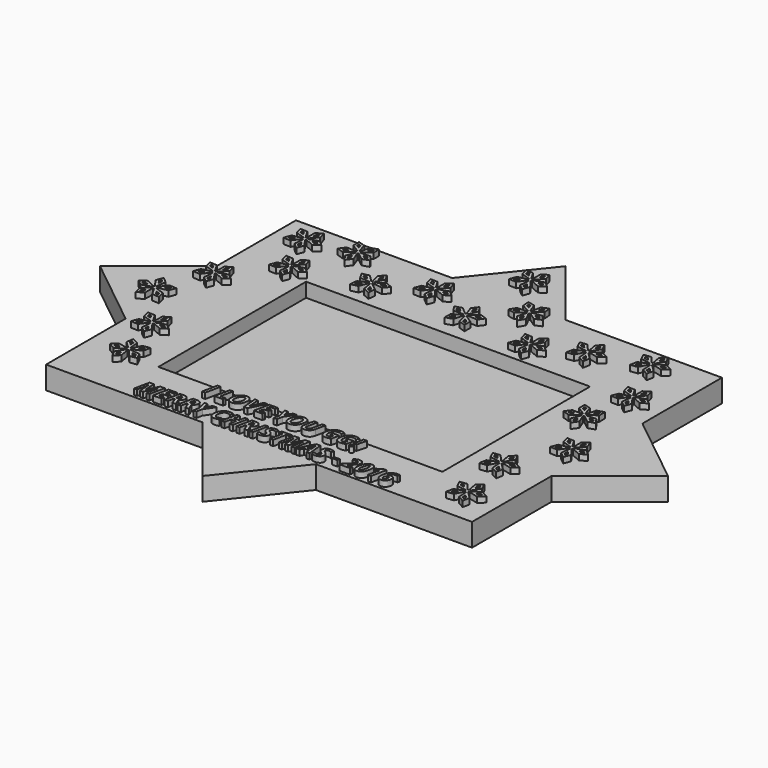
from build123d import *

# Parameters (mm, degrees)
F1_DEPTH     = 4
F4_W         = 100
F4_H         = 65
F5_DEPTH     = 5
F6_DEPTH     = 2
F7_TEXT_SIZE = 7.546576527
F8_DEPTH     = 2


# Not quite as in the source:
# - Text() gives the source's letters only with a copy of the font that has no kerning and outlines rounded to 1/6400 em; it was checked with that copy


with BuildPart() as f1:
    # F0 (on Top) → F1 (new body, symmetric)
    with BuildSketch(Plane.XY):
        Polygon((75, 20), (75, 55), (20, 55), (0, 80), (-20, 55), (-75, 55), (-75, 20), (-100, 0), (-75, -20), (-75, -55), (-20, -55), (0, -80), (20, -55), (75, -55), (75, -20), (100, 0), align=None)
    extrude(amount=F1_DEPTH, both=True)

    # F4 (on face) → F5 (cut)
    with BuildSketch(Plane.XY.offset(4)):
        with Locations((0, -4.2958769202)):
            Rectangle(F4_W, F4_H)
    extrude(amount=-F5_DEPTH, mode=Mode.SUBTRACT)

    # F2 (on face) → F6 (join)
    with BuildSketch(Plane.XY.offset(4)):
        with BuildLine():
            Line((63.1994701679, 31.4178951368), (60.6442793174, 31.5524958216))
            Line((60.6442793174, 31.5524958216), (61.3153708432, 29.0833352779))
            Line((61.3153708432, 29.0833352779), (64.6001066479, 28.016059918))
            ThreePointArc((64.6001066479, 28.016059918), (64.5643629359, 27.8223093015), (64.5803085929, 27.6259355498))
            Line((64.5803085929, 27.6259355498), (61.2044020685, 26.8966748697))
            Line((61.2044020685, 26.8966748697), (60.2867918134, 24.5081378601))
            Line((60.2867918134, 24.5081378601), (62.8424817245, 24.3833712589))
            Line((62.8424817245, 24.3833712589), (64.8725600959, 27.1775344264))
            ThreePointArc((64.8725600959, 27.1775344264), (65.0457824678, 27.083667903), (65.237472483, 27.0381502975))
            Line((65.237472483, 27.0381502975), (64.8878281174, 23.6021184556))
            Line((64.8878281174, 23.6021184556), (66.8759046418, 21.9913207154))
            Line((66.8759046418, 21.9913207154), (67.7843163458, 24.3833712589))
            Line((67.7843163458, 24.3833712589), (65.7542379744, 27.1775344264))
            ThreePointArc((65.7542379744, 27.1775344264), (65.8970389999, 27.313272341), (65.9995642876, 27.4815146655))
            Line((65.9995642876, 27.4815146655), (69.15937871, 26.0871908808))
            Line((69.15937871, 26.0871908808), (71.3056878294, 27.480200138))
            Line((71.3056878294, 27.480200138), (69.3114272272, 29.0833352779))
            Line((69.3114272272, 29.0833352779), (66.0266914224, 28.016059918))
            ThreePointArc((66.0266914224, 28.016059918), (65.9417249379, 28.1938170862), (65.8133990352, 28.3433141666))
            Line((65.8133990352, 28.3433141666), (68.115916112, 30.9176065182))
            Line((68.115916112, 30.9176065182), (67.4543315738, 33.389331326))
            Line((67.4543315738, 33.389331326), (65.3133990352, 31.9880727875))
            Line((65.3133990352, 31.9880727875), (65.3133990352, 28.5342971722))
            ThreePointArc((65.3133990352, 28.5342971722), (65.1180858343, 28.5084192293), (64.9362507771, 28.4325711818))
            Line((64.9362507771, 28.4325711818), (63.1994701679, 31.4178951368))
        make_face()
        Polygon((66.8188202697, 24.1229536578), (66.5160163683, 23.3256034766), (65.8533241935, 23.8625360567), (65.9951811661, 25.2565956289), align=None, mode=Mode.SUBTRACT)
        Polygon((62.2964551725, 25.2211391292), (61.4445585355, 25.2627279962), (61.7504286205, 26.0589069994), (63.1200942761, 26.3547811003), align=None, mode=Mode.SUBTRACT)
        Polygon((61.9434039514, 29.8615218975), (61.7197067761, 30.6845754121), (62.5714370596, 30.6397085171), (63.2760800154, 29.4285091956), align=None, mode=Mode.SUBTRACT)
        Polygon((66.2475713941, 31.6312506978), (66.9612155737, 32.0983368772), (67.1817437531, 31.274428608), (66.2475713941, 30.2299921593), align=None, mode=Mode.SUBTRACT)
        Polygon((69.2607769989, 28.0852630793), (69.9263859742, 27.5501970319), (69.2100289384, 27.0852630793), (67.9263859742, 27.6516931529), align=None, mode=Mode.SUBTRACT)
        with BuildLine():
            Line((60.4743340463, 15.1066376163), (58.0410464334, 15.89798395))
            Line((58.0410464334, 15.89798395), (58.0502052958, 13.3392667437))
            Line((58.0502052958, 13.3392667437), (60.9467852527, 11.4582057254))
            ThreePointArc((60.9467852527, 11.4582057254), (60.8621131286, 11.2803081545), (60.8266901836, 11.0864986364))
            Line((60.8266901836, 11.0864986364), (57.3770683317, 11.2558358144))
            Line((57.3770683317, 11.2558358144), (55.8725260198, 9.1861812398))
            Line((55.8725260198, 9.1861812398), (58.3088409363, 8.404204735))
            Line((58.3088409363, 8.404204735), (60.9929287076, 10.5777361558))
            ThreePointArc((60.9929287076, 10.5777361558), (61.1359542263, 10.4422348077), (61.3093317395, 10.3486551503))
            Line((61.3093317395, 10.3486551503), (60.0822907364, 7.1201978751))
            Line((60.0822907364, 7.1201978751), (61.585720063, 5.0497346693))
            Line((61.585720063, 5.0497346693), (63.0822866263, 7.1251638173))
            Line((63.0822866263, 7.1251638173), (61.8445641408, 10.3495411293))
            ThreePointArc((61.8445641408, 10.3495411293), (62.0176308968, 10.4436942615), (62.1602070378, 10.5796683707))
            Line((62.1602070378, 10.5796683707), (64.8514758442, 8.4150348653))
            Line((64.8514758442, 8.4150348653), (67.2851885796, 9.2050728063))
            Line((67.2851885796, 9.2050728063), (65.7738026656, 11.2697350658))
            Line((65.7738026656, 11.2697350658), (62.3247603297, 11.0889784163))
            ThreePointArc((62.3247603297, 11.0889784163), (62.2886959485, 11.2826696003), (62.2034353365, 11.4602858788))
            Line((62.2034353365, 11.4602858788), (65.0937719348, 13.3509260745))
            Line((65.0937719348, 13.3509260745), (65.0944597975, 15.9096595802))
            Line((65.0944597975, 15.9096595802), (62.6638053693, 15.1102618839))
            Line((62.6638053693, 15.1102618839), (61.7699024625, 11.7741708188))
            ThreePointArc((61.7699024625, 11.7741708188), (61.5745466931, 11.7997254216), (61.379276596, 11.7735242095))
            Line((61.379276596, 11.7735242095), (60.4743340463, 15.1066376163))
        make_face()
        Polygon((62.0822879963, 7.1235085032), (61.5834324752, 6.4316987872), (61.0822893664, 7.1218531892), (61.5801218471, 8.4316960472), align=None, mode=Mode.SUBTRACT)
        Polygon((57.9982500681, 9.3547484281), (57.1861450959, 9.6154072631), (57.6876591999, 10.3052921213), (59.0872324822, 10.2365889995), align=None, mode=Mode.SUBTRACT)
        Polygon((65.4665582086, 10.3187805964), (65.9710018247, 9.6296742031), (65.1587203012, 9.3659893347), (64.0654193012, 10.2453500178), align=None, mode=Mode.SUBTRACT)
        Polygon((58.8582482127, 13.9283903679), (58.8551952585, 14.7812961033), (59.6662911295, 14.5175139921), (60.0334425069, 13.1652102697), align=None, mode=Mode.SUBTRACT)
        Polygon((63.4737942244, 14.5238166141), (64.2840123672, 14.7902825129), (64.2837830796, 13.9373713443), (63.1111218276, 13.1703048025), align=None, mode=Mode.SUBTRACT)
        with BuildLine():
            Line((54.531646123, 49.5059511711), (51.9919011994, 49.1948027344))
            Line((51.9919011994, 49.1948027344), (53.0815625657, 46.879688108))
            Line((53.0815625657, 46.879688108), (56.5017262742, 46.3990154456))
            ThreePointArc((56.5017262742, 46.3990154456), (56.5001700309, 46.2020015058), (56.5499733817, 46.0113800469))
            Line((56.5499733817, 46.0113800469), (53.3519892511, 44.7069784593))
            Line((53.3519892511, 44.7069784593), (52.8630846567, 42.1953873453))
            Line((52.8630846567, 42.1953873453), (55.4016133884, 42.5163071248))
            Line((55.4016133884, 42.5163071248), (56.9156489656, 45.6205400851))
            ThreePointArc((56.9156489656, 45.6205400851), (57.1025394512, 45.5581793543), (57.2992213136, 45.5466398853))
            Line((57.2992213136, 45.5466398853), (57.5515494993, 42.1020939809))
            Line((57.5515494993, 42.1020939809), (59.7891347663, 40.8609937433))
            Line((59.7891347663, 40.8609937433), (60.2683704375, 43.3744477011))
            Line((60.2683704375, 43.3744477011), (57.783932176, 45.773641842))
            ThreePointArc((57.783932176, 45.773641842), (57.9009930915, 45.9321147305), (57.9727458167, 46.1156044054))
            Line((57.9727458167, 46.1156044054), (61.3266773423, 45.2911595482))
            Line((61.3266773423, 45.2911595482), (63.1984856844, 47.035708532))
            Line((63.1984856844, 47.035708532), (60.9561408862, 48.2681887276))
            Line((60.9561408862, 48.2681887276), (57.9066380204, 46.6467392919))
            ThreePointArc((57.9066380204, 46.6467392919), (57.7920951594, 46.8070416542), (57.6397589199, 46.9319839788))
            Line((57.6397589199, 46.9319839788), (59.460274413, 49.8669949397))
            Line((59.460274413, 49.8669949397), (58.3795303219, 52.1862857442))
            Line((58.3795303219, 52.1862857442), (56.5144493508, 50.4345464378))
            Line((56.5144493508, 50.4345464378), (57.1141911925, 47.0332414346))
            ThreePointArc((57.1141911925, 47.0332414346), (56.9263388957, 46.9738408544), (56.7604371968, 46.8675697828))
            Line((56.7604371968, 46.8675697828), (54.531646123, 49.5059511711))
        make_face()
        Polygon((54.7184053426, 43.246530903), (53.8722290987, 43.1395576431), (54.0351972969, 43.9767546812), (55.3326766551, 44.5059737347), align=None, mode=Mode.SUBTRACT)
        Polygon((53.5649237515, 47.755109129), (53.201703296, 48.5268140045), (54.0482849372, 48.6305301501), (54.9525453381, 47.560091633), align=None, mode=Mode.SUBTRACT)
        Polygon((59.3627634581, 42.9503297944), (59.2030182344, 42.1125118084), (58.4571564787, 42.5262118876), (58.3547824209, 43.9237257673), align=None, mode=Mode.SUBTRACT)
        Polygon((61.0795735671, 47.2764841685), (61.8279836906, 46.8651287623), (61.2032446614, 46.2828641073), (59.8407435681, 46.6177865738), align=None, mode=Mode.SUBTRACT)
        Polygon((57.4963910382, 50.2453626051), (58.1180846952, 50.8292757072), (58.4783327256, 50.0561787724), (57.7397170299, 48.8653923324), align=None, mode=Mode.SUBTRACT)
        with BuildLine():
            Line((69.176194365, -2.7749478988), (66.6210035146, -2.640347214))
            Line((66.6210035146, -2.640347214), (67.2920950403, -5.1095077577))
            Line((67.2920950403, -5.1095077577), (70.5768308451, -6.1767831176))
            ThreePointArc((70.5768308451, -6.1767831176), (70.5410871331, -6.3705337341), (70.5570327901, -6.5669074858))
            Line((70.5570327901, -6.5669074858), (67.1811262657, -7.2961681658))
            Line((67.1811262657, -7.2961681658), (66.2635160106, -9.6847051755))
            Line((66.2635160106, -9.6847051755), (68.8192059217, -9.8094717767))
            Line((68.8192059217, -9.8094717767), (70.8492842931, -7.0153086091))
            ThreePointArc((70.8492842931, -7.0153086091), (71.022506665, -7.1091751326), (71.2141966802, -7.1546927381))
            Line((71.2141966802, -7.1546927381), (70.8645523146, -10.59072458))
            Line((70.8645523146, -10.59072458), (72.852628839, -12.2015223202))
            Line((72.852628839, -12.2015223202), (73.761040543, -9.8094717767))
            Line((73.761040543, -9.8094717767), (71.7309621716, -7.0153086091))
            ThreePointArc((71.7309621716, -7.0153086091), (71.8737631971, -6.8795706945), (71.9762884848, -6.7113283701))
            Line((71.9762884848, -6.7113283701), (75.1361029072, -8.1056521548))
            Line((75.1361029072, -8.1056521548), (77.2824120266, -6.7126428976))
            Line((77.2824120266, -6.7126428976), (75.2881514244, -5.1095077577))
            Line((75.2881514244, -5.1095077577), (72.0034156196, -6.1767831176))
            ThreePointArc((72.0034156196, -6.1767831176), (71.9184491351, -5.9990259494), (71.7901232323, -5.849528869))
            Line((71.7901232323, -5.849528869), (74.0926403092, -3.2752365174))
            Line((74.0926403092, -3.2752365174), (73.431055771, -0.8035117096))
            Line((73.431055771, -0.8035117096), (71.2901232323, -2.204770248))
            Line((71.2901232323, -2.204770248), (71.2901232323, -5.6585458634))
            ThreePointArc((71.2901232323, -5.6585458634), (71.0948100315, -5.6844238063), (70.9129749743, -5.7602718538))
            Line((70.9129749743, -5.7602718538), (69.176194365, -2.7749478988))
        make_face()
        Polygon((72.7955444668, -10.0698893778), (72.4927405655, -10.867239559), (71.8300483907, -10.3303069789), (71.9719053633, -8.9362474067), align=None, mode=Mode.SUBTRACT)
        Polygon((68.2731793697, -8.9717039064), (67.4212827327, -8.9301150393), (67.7271528177, -8.1339360361), (69.0968184732, -7.8380619353), align=None, mode=Mode.SUBTRACT)
        Polygon((75.237501196, -6.1075799563), (75.9031101714, -6.6426460036), (75.1867531355, -7.1075799563), (73.9031101714, -6.5411498826), align=None, mode=Mode.SUBTRACT)
        Polygon((67.9201281486, -4.3313211381), (67.6964309733, -3.5082676235), (68.5481612568, -3.5531345184), (69.2528042126, -4.76433384), align=None, mode=Mode.SUBTRACT)
        Polygon((72.2242955913, -2.5615923378), (72.9379397709, -2.0945061583), (73.1584679503, -2.9184144276), (72.2242955913, -3.9628508763), align=None, mode=Mode.SUBTRACT)
        with BuildLine():
            Line((58.7020704823, -22.0312884666), (56.1623255587, -22.3424369034))
            Line((56.1623255587, -22.3424369034), (57.2519869251, -24.6575515297))
            Line((57.2519869251, -24.6575515297), (60.6721506335, -25.1382241921))
            ThreePointArc((60.6721506335, -25.1382241921), (60.6705943902, -25.3352381319), (60.720397741, -25.5258595908))
            Line((60.720397741, -25.5258595908), (57.5224136105, -26.8302611784))
            Line((57.5224136105, -26.8302611784), (57.033509016, -29.3418522924))
            Line((57.033509016, -29.3418522924), (59.5720377477, -29.0209325129))
            Line((59.5720377477, -29.0209325129), (61.086073325, -25.9166995526))
            ThreePointArc((61.086073325, -25.9166995526), (61.2729638106, -25.9790602834), (61.469645673, -25.9905997524))
            Line((61.469645673, -25.9905997524), (61.7219738586, -29.4351456568))
            Line((61.7219738586, -29.4351456568), (63.9595591256, -30.6762458944))
            Line((63.9595591256, -30.6762458944), (64.4387947969, -28.1627919366))
            Line((64.4387947969, -28.1627919366), (61.9543565353, -25.7635977957))
            ThreePointArc((61.9543565353, -25.7635977957), (62.0714174509, -25.6051249072), (62.143170176, -25.4216352323))
            Line((62.143170176, -25.4216352323), (65.4971017016, -26.2460800895))
            Line((65.4971017016, -26.2460800895), (67.3689100438, -24.5015311057))
            Line((67.3689100438, -24.5015311057), (65.1265652456, -23.2690509101))
            Line((65.1265652456, -23.2690509101), (62.0770623797, -24.8905003458))
            ThreePointArc((62.0770623797, -24.8905003458), (61.9625195187, -24.7301979835), (61.8101832792, -24.6052556589))
            Line((61.8101832792, -24.6052556589), (63.6306987723, -21.670244698))
            Line((63.6306987723, -21.670244698), (62.5499546812, -19.3509538935))
            Line((62.5499546812, -19.3509538935), (60.6848737102, -21.1026932))
            Line((60.6848737102, -21.1026932), (61.2846155518, -24.5039982031))
            ThreePointArc((61.2846155518, -24.5039982031), (61.096763255, -24.5633987833), (60.9308615561, -24.6696698549))
            Line((60.9308615561, -24.6696698549), (58.7020704823, -22.0312884666))
        make_face()
        Polygon((58.888829702, -28.2907087347), (58.0426534581, -28.3976819946), (58.2056216562, -27.5604849566), (59.5031010144, -27.031265903), align=None, mode=Mode.SUBTRACT)
        Polygon((63.5331878175, -28.5869098433), (63.3734425937, -29.4247278293), (62.627580838, -29.0110277501), (62.5252067802, -27.6135138704), align=None, mode=Mode.SUBTRACT)
        Polygon((65.2499979265, -24.2607554692), (65.99840805, -24.6721108754), (65.3736690207, -25.2543755304), (64.0111679275, -24.9194530639), align=None, mode=Mode.SUBTRACT)
        Polygon((57.7353481108, -23.7821305087), (57.3721276554, -23.0104256332), (58.2187092966, -22.9067094876), (59.1229696975, -23.9771480047), align=None, mode=Mode.SUBTRACT)
        Polygon((61.6668153975, -21.2918770327), (62.2885090546, -20.7079639305), (62.6487570849, -21.4810608653), (61.9101413892, -22.6718473053), align=None, mode=Mode.SUBTRACT)
        with BuildLine():
            Line((62.2558930258, -41.1344152125), (59.7161481023, -41.4455636493))
            Line((59.7161481023, -41.4455636493), (60.8058094686, -43.7606782757))
            Line((60.8058094686, -43.7606782757), (64.225973177, -44.2413509381))
            ThreePointArc((64.225973177, -44.2413509381), (64.2244169338, -44.4383648779), (64.2742202845, -44.6289863368))
            Line((64.2742202845, -44.6289863368), (61.076236154, -45.9333879244))
            Line((61.076236154, -45.9333879244), (60.5873315596, -48.4449790384))
            Line((60.5873315596, -48.4449790384), (63.1258602913, -48.1240592589))
            Line((63.1258602913, -48.1240592589), (64.6398958685, -45.0198262986))
            ThreePointArc((64.6398958685, -45.0198262986), (64.8267863541, -45.0821870294), (65.0234682165, -45.0937264984))
            Line((65.0234682165, -45.0937264984), (65.2757964021, -48.5382724028))
            Line((65.2757964021, -48.5382724028), (67.5133816691, -49.7793726404))
            Line((67.5133816691, -49.7793726404), (67.9926173404, -47.2659186826))
            Line((67.9926173404, -47.2659186826), (65.5081790789, -44.8667245417))
            ThreePointArc((65.5081790789, -44.8667245417), (65.6252399944, -44.7082516532), (65.6969927195, -44.5247619783))
            Line((65.6969927195, -44.5247619783), (69.0509242452, -45.3492068355))
            Line((69.0509242452, -45.3492068355), (70.9227325873, -43.6046578517))
            Line((70.9227325873, -43.6046578517), (68.6803877891, -42.3721776561))
            Line((68.6803877891, -42.3721776561), (65.6308849232, -43.9936270918))
            ThreePointArc((65.6308849232, -43.9936270918), (65.5163420622, -43.8333247295), (65.3640058227, -43.7083824049))
            Line((65.3640058227, -43.7083824049), (67.1845213159, -40.773371444))
            Line((67.1845213159, -40.773371444), (66.1037772248, -38.4540806395))
            Line((66.1037772248, -38.4540806395), (64.2386962537, -40.2058199459))
            Line((64.2386962537, -40.2058199459), (64.8384380953, -43.6071249491))
            ThreePointArc((64.8384380953, -43.6071249491), (64.6505857985, -43.6665255293), (64.4846840997, -43.7727966009))
            Line((64.4846840997, -43.7727966009), (62.2558930258, -41.1344152125))
        make_face()
        Polygon((62.4426522455, -47.3938354807), (61.5964760016, -47.5008087405), (61.7594441997, -46.6636117025), (63.0569235579, -46.134392649), align=None, mode=Mode.SUBTRACT)
        Polygon((67.087010361, -47.6900365893), (66.9272651372, -48.5278545752), (66.1814033816, -48.1141544961), (66.0790293237, -46.7166406164), align=None, mode=Mode.SUBTRACT)
        Polygon((61.2891706543, -42.8852572547), (60.9259501989, -42.1135523792), (61.7725318401, -42.0098362336), (62.676792241, -43.0802747507), align=None, mode=Mode.SUBTRACT)
        Polygon((68.80382047, -43.3638822152), (69.5522305935, -43.7752376214), (68.9274915642, -44.3575022764), (67.564990471, -44.0225798099), align=None, mode=Mode.SUBTRACT)
        Polygon((65.2206379411, -40.3950037786), (65.8423315981, -39.8110906765), (66.2025796285, -40.5841876113), (65.4639639327, -41.7749740513), align=None, mode=Mode.SUBTRACT)
        with BuildLine():
            Line((36.2130666452, 44.3193224602), (33.6733217216, 44.0081740234))
            Line((33.6733217216, 44.0081740234), (34.7629830879, 41.693059397))
            Line((34.7629830879, 41.693059397), (38.1831467964, 41.2123867346))
            ThreePointArc((38.1831467964, 41.2123867346), (38.1815905531, 41.0153727949), (38.2313939039, 40.824751336))
            Line((38.2313939039, 40.824751336), (35.0334097734, 39.5203497484))
            Line((35.0334097734, 39.5203497484), (34.5445051789, 37.0087586343))
            Line((34.5445051789, 37.0087586343), (37.0830339106, 37.3296784138))
            Line((37.0830339106, 37.3296784138), (38.5970694879, 40.4339113742))
            ThreePointArc((38.5970694879, 40.4339113742), (38.7839599734, 40.3715506433), (38.9806418359, 40.3600111743))
            Line((38.9806418359, 40.3600111743), (39.2329700215, 36.9154652699))
            Line((39.2329700215, 36.9154652699), (41.4705552885, 35.6743650324))
            Line((41.4705552885, 35.6743650324), (41.9497909598, 38.1878189902))
            Line((41.9497909598, 38.1878189902), (39.4653526982, 40.587013131))
            ThreePointArc((39.4653526982, 40.587013131), (39.5824136138, 40.7454860196), (39.6541663389, 40.9289756944))
            Line((39.6541663389, 40.9289756944), (43.0080978645, 40.1045308373))
            Line((43.0080978645, 40.1045308373), (44.8799062067, 41.8490798211))
            Line((44.8799062067, 41.8490798211), (42.6375614084, 43.0815600166))
            Line((42.6375614084, 43.0815600166), (39.5880585426, 41.460110581))
            ThreePointArc((39.5880585426, 41.460110581), (39.4735156816, 41.6204129432), (39.3211794421, 41.7453552678))
            Line((39.3211794421, 41.7453552678), (41.1416949352, 44.6803662287))
            Line((41.1416949352, 44.6803662287), (40.0609508441, 46.9996570333))
            Line((40.0609508441, 46.9996570333), (38.195869873, 45.2479177268))
            Line((38.195869873, 45.2479177268), (38.7956117147, 41.8466127236))
            ThreePointArc((38.7956117147, 41.8466127236), (38.6077594179, 41.7872121434), (38.441857719, 41.6809410719))
            Line((38.441857719, 41.6809410719), (36.2130666452, 44.3193224602))
        make_face()
        Polygon((36.3998258649, 38.059902192), (35.553649621, 37.9529289322), (35.7166178191, 38.7901259702), (37.0140971773, 39.3193450237), align=None, mode=Mode.SUBTRACT)
        Polygon((41.0441839804, 37.7637010834), (40.8844387566, 36.9258830975), (40.1385770009, 37.3395831767), (40.0362029431, 38.7370970563), align=None, mode=Mode.SUBTRACT)
        Polygon((35.2463442737, 42.5684804181), (34.8831238183, 43.3401852935), (35.7297054595, 43.4439014391), (36.6339658604, 42.373462922), align=None, mode=Mode.SUBTRACT)
        Polygon((42.7609940894, 42.0898554576), (43.5094042129, 41.6785000513), (42.8846651836, 41.0962353963), (41.5221640904, 41.4311578629), align=None, mode=Mode.SUBTRACT)
        Polygon((39.1778115604, 45.0587338941), (39.7995052175, 45.6426469963), (40.1597532478, 44.8695500614), (39.4211375521, 43.6787636215), align=None, mode=Mode.SUBTRACT)
        with BuildLine():
            Line((-2.0873219995, 68.2391146027), (-4.6425128499, 68.3737152875))
            Line((-4.6425128499, 68.3737152875), (-3.9714213242, 65.9045547438))
            Line((-3.9714213242, 65.9045547438), (-0.6866855194, 64.8372793839))
            ThreePointArc((-0.6866855194, 64.8372793839), (-0.7224292314, 64.6435287674), (-0.7064835744, 64.4471550157))
            Line((-0.7064835744, 64.4471550157), (-4.0823900988, 63.7178943357))
            Line((-4.0823900988, 63.7178943357), (-5.0000003539, 61.329357326))
            Line((-5.0000003539, 61.329357326), (-2.4443104428, 61.2045907248))
            Line((-2.4443104428, 61.2045907248), (-0.4142320714, 63.9987538923))
            ThreePointArc((-0.4142320714, 63.9987538923), (-0.2410096995, 63.9048873689), (-0.0493196843, 63.8593697634))
            Line((-0.0493196843, 63.8593697634), (-0.3989640499, 60.4233379215))
            Line((-0.3989640499, 60.4233379215), (1.5891124745, 58.8125401813))
            Line((1.5891124745, 58.8125401813), (2.4975241785, 61.2045907248))
            Line((2.4975241785, 61.2045907248), (0.4674458071, 63.9987538923))
            ThreePointArc((0.4674458071, 63.9987538923), (0.6102468326, 64.1344918069), (0.7127721203, 64.3027341314))
            Line((0.7127721203, 64.3027341314), (3.8725865427, 62.9084103467))
            Line((3.8725865427, 62.9084103467), (6.0188956621, 64.3014196039))
            Line((6.0188956621, 64.3014196039), (4.0246350599, 65.9045547438))
            Line((4.0246350599, 65.9045547438), (0.7398992551, 64.8372793839))
            ThreePointArc((0.7398992551, 64.8372793839), (0.6549327706, 65.0150365521), (0.5266068679, 65.1645336325))
            Line((0.5266068679, 65.1645336325), (2.8291239447, 67.7388259841))
            Line((2.8291239447, 67.7388259841), (2.1675394065, 70.2105507919))
            Line((2.1675394065, 70.2105507919), (0.0266068679, 68.8092922535))
            Line((0.0266068679, 68.8092922535), (0.0266068679, 65.3555166381))
            ThreePointArc((0.0266068679, 65.3555166381), (-0.168706333, 65.3296386952), (-0.3505413902, 65.2537906477))
            Line((-0.3505413902, 65.2537906477), (-2.0873219995, 68.2391146027))
        make_face()
        Polygon((-2.9903369948, 62.0423585951), (-3.8422336318, 62.0839474622), (-3.5363635468, 62.8801264654), (-2.1666978913, 63.1760005662), align=None, mode=Mode.SUBTRACT)
        Polygon((1.5320281024, 60.9441731237), (1.229224201, 60.1468229425), (0.5665320262, 60.6837555226), (0.7083889988, 62.0778150948), align=None, mode=Mode.SUBTRACT)
        Polygon((3.9739848315, 64.9064825452), (4.6395938069, 64.3714164979), (3.923236771, 63.9064825452), (2.6395938069, 64.4729126189), align=None, mode=Mode.SUBTRACT)
        Polygon((-3.3433882159, 66.6827413634), (-3.5670853912, 67.505794878), (-2.7153551077, 67.4609279831), (-2.0107121519, 66.2497286615), align=None, mode=Mode.SUBTRACT)
        Polygon((0.9607792268, 68.4524701637), (1.6744234064, 68.9195563432), (1.8949515858, 68.0956480739), (0.9607792268, 67.0512116252), align=None, mode=Mode.SUBTRACT)
        with BuildLine():
            Line((10.203743278, 53.3324640832), (7.7107446817, 53.908724116))
            Line((7.7107446817, 53.908724116), (7.9428755905, 51.3605418486))
            Line((7.9428755905, 51.3605418486), (10.9923784563, 49.7390924129))
            ThreePointArc((10.9923784563, 49.7390924129), (10.9235333301, 49.5544921341), (10.9051367926, 49.3583328066))
            Line((10.9051367926, 49.3583328066), (7.4538830858, 49.2263712509))
            Line((7.4538830858, 49.2263712509), (6.1354482933, 47.0334628341))
            Line((6.1354482933, 47.0334628341), (8.6306460392, 46.4668008221))
            Line((8.6306460392, 46.4668008221), (11.1150843007, 48.865994963))
            ThreePointArc((11.1150843007, 48.865994963), (11.2693752848, 48.7434747338), (11.4502490487, 48.6653620211))
            Line((11.4502490487, 48.6653620211), (10.5092558989, 45.3422463305))
            Line((10.5092558989, 45.3422463305), (12.1874169815, 43.410694362))
            Line((12.1874169815, 43.410694362), (13.4974030883, 45.6086602458))
            Line((13.4974030883, 45.6086602458), (11.9833675111, 48.7128932061))
            ThreePointArc((11.9833675111, 48.7128932061), (12.1475697096, 48.821771819), (12.2777523809, 48.9696548351))
            Line((12.2777523809, 48.9696548351), (15.1474403379, 47.0478179455))
            Line((15.1474403379, 47.0478179455), (17.503035718, 48.0469615947))
            Line((17.503035718, 48.0469615947), (15.817453911, 49.972041229))
            Line((15.817453911, 49.972041229), (12.3972902025, 49.4913685666))
            ThreePointArc((12.3972902025, 49.4913685666), (12.3444817582, 49.6811794792), (12.2440653098, 49.8506889221))
            Line((12.2440653098, 49.8506889221), (14.9586231542, 51.9860440941))
            Line((14.9586231542, 51.9860440941), (14.7363000803, 54.5351007975))
            Line((14.7363000803, 54.5351007975), (12.3845671259, 53.5268995588))
            Line((12.3845671259, 53.5268995588), (11.7848252842, 50.1255945556))
            ThreePointArc((11.7848252842, 50.1255945556), (11.5879856721, 50.1340255382), (11.3957422228, 50.0909051192))
            Line((11.3957422228, 50.0909051192), (10.203743278, 53.3324640832))
        make_face()
        Polygon((12.5013540252, 45.5198556074), (12.0646919895, 44.7872003128), (11.505304962, 45.431050969), (11.8870827127, 46.7792984391), align=None, mode=Mode.SUBTRACT)
        Polygon((8.2383917214, 47.3866576317), (7.4066591394, 47.5755449691), (7.8461374036, 48.3065144413), (9.2463727586, 48.3600536046), align=None, mode=Mode.SUBTRACT)
        Polygon((15.594259755, 48.9979273096), (16.1568433904, 48.3554083322), (15.3706344939, 48.0219318648), (14.2048525008, 48.8026588544), align=None, mode=Mode.SUBTRACT)
        Polygon((8.696498153, 52.0178492601), (8.6191211834, 52.8672433492), (9.4501207155, 52.6751566717), (9.9337360065, 51.3599982242), align=None, mode=Mode.SUBTRACT)
        Polygon((13.242585802, 53.0132810705), (14.0264967868, 53.3493481501), (14.1006044781, 52.4996625823), (12.9992598104, 51.6333107979), align=None, mode=Mode.SUBTRACT)
        with BuildLine():
            Line((-4.2115295507, 39.8939389404), (-6.6586596831, 39.1464954698))
            Line((-6.6586596831, 39.1464954698), (-5.1835372855, 37.0557703471))
            Line((-5.1835372855, 37.0557703471), (-1.7318656169, 37.1763053778))
            ThreePointArc((-1.7318656169, 37.1763053778), (-1.6991871057, 36.9820142837), (-1.6170393108, 36.8029370542))
            Line((-1.6170393108, 36.8029370542), (-4.539931918, 34.9630281412))
            Line((-4.539931918, 34.9630281412), (-4.585275733, 32.4046963479))
            Line((-4.585275733, 32.4046963479), (-2.1410400917, 33.161551523))
            Line((-2.1410400917, 33.161551523), (-1.1890505135, 36.4815337284))
            ThreePointArc((-1.1890505135, 36.4815337284), (-0.9941704871, 36.4525735895), (-0.7984728563, 36.4753628779))
            Line((-0.7984728563, 36.4753628779), (0.0481610164, 33.1269636952))
            Line((0.0481610164, 33.1269636952), (2.4672671299, 32.293271163))
            Line((2.4672671299, 32.293271163), (2.5027654351, 34.8517585085))
            Line((2.5027654351, 34.8517585085), (-0.3605443172, 36.7830853228))
            ThreePointArc((-0.3605443172, 36.7830853228), (-0.2727803483, 36.9594780667), (-0.233980356, 37.1526398511))
            Line((-0.233980356, 37.1526398511), (3.2121607606, 36.9231242612))
            Line((3.2121607606, 36.9231242612), (4.7525943762, 38.9662057335))
            Line((4.7525943762, 38.9662057335), (2.330297894, 39.7905826976))
            Line((2.330297894, 39.7905826976), (-0.3913144314, 37.6642261069))
            ThreePointArc((-0.3913144314, 37.6642261069), (-0.5319533421, 37.8022029569), (-0.7036712588, 37.8987942165))
            Line((-0.7036712588, 37.8987942165), (0.5795272085, 41.1053449638))
            Line((0.5795272085, 41.1053449638), (-0.8875385731, 43.2017312876))
            Line((-0.8875385731, 43.2017312876), (-2.4200984351, 41.1527369255))
            Line((-2.4200984351, 41.1527369255), (-1.2388376041, 37.907249466))
            ThreePointArc((-1.2388376041, 37.907249466), (-1.4135212, 37.816131105), (-1.5584487013, 37.6826660021))
            Line((-1.5584487013, 37.6826660021), (-4.2115295507, 39.8939389404))
        make_face()
        Polygon((-4.8595347072, 38.0018265449), (-5.3512421731, 38.6987349191), (-4.535532129, 38.9478827426), (-3.4591297776, 38.0507297626), align=None, mode=Mode.SUBTRACT)
        Polygon((-2.9406707005, 33.7620437291), (-3.7554159142, 33.5097586707), (-3.7403013092, 34.3625359352), (-2.5544315021, 35.1090198882), align=None, mode=Mode.SUBTRACT)
        Polygon((1.6845639622, 34.2768269041), (1.6727311938, 33.4239977889), (0.8663624893, 33.7018952997), (0.5228679849, 35.0604007347), align=None, mode=Mode.SUBTRACT)
        Polygon((2.6240630446, 38.8353782193), (3.4325342533, 38.5602322801), (2.91839561, 37.8783287396), (1.5184352939, 37.9715671494), align=None, mode=Mode.SUBTRACT)
        Polygon((-1.4202232206, 41.1369396049), (-0.9093699332, 41.8199377256), (-0.420348006, 41.1211422844), (-0.9409645744, 39.8201872966), align=None, mode=Mode.SUBTRACT)
        with BuildLine():
            Line((-19.2796059392, 47.6930219819), (-21.8347967896, 47.8276226667))
            Line((-21.8347967896, 47.8276226667), (-21.1637052639, 45.358462123))
            Line((-21.1637052639, 45.358462123), (-17.8789694591, 44.2911867631))
            ThreePointArc((-17.8789694591, 44.2911867631), (-17.9147131711, 44.0974361466), (-17.8987675141, 43.9010623949))
            Line((-17.8987675141, 43.9010623949), (-21.2746740385, 43.1718017149))
            Line((-21.2746740385, 43.1718017149), (-22.1922842936, 40.7832647052))
            Line((-22.1922842936, 40.7832647052), (-19.6365943825, 40.658498104))
            Line((-19.6365943825, 40.658498104), (-17.6065160111, 43.4526612716))
            ThreePointArc((-17.6065160111, 43.4526612716), (-17.4332936392, 43.3587947481), (-17.241603624, 43.3132771426))
            Line((-17.241603624, 43.3132771426), (-17.5912479896, 39.8772453007))
            Line((-17.5912479896, 39.8772453007), (-15.6031714652, 38.2664475605))
            Line((-15.6031714652, 38.2664475605), (-14.6947597612, 40.658498104))
            Line((-14.6947597612, 40.658498104), (-16.7248381326, 43.4526612716))
            ThreePointArc((-16.7248381326, 43.4526612716), (-16.5820371071, 43.5883991862), (-16.4795118194, 43.7566415106))
            Line((-16.4795118194, 43.7566415106), (-13.319697397, 42.3623177259))
            Line((-13.319697397, 42.3623177259), (-11.1733882776, 43.7553269831))
            Line((-11.1733882776, 43.7553269831), (-13.1676488798, 45.358462123))
            Line((-13.1676488798, 45.358462123), (-16.4523846846, 44.2911867631))
            ThreePointArc((-16.4523846846, 44.2911867631), (-16.5373511691, 44.4689439313), (-16.6656770719, 44.6184410117))
            Line((-16.6656770719, 44.6184410117), (-14.363159995, 47.1927333633))
            Line((-14.363159995, 47.1927333633), (-15.0247445332, 49.6644581711))
            Line((-15.0247445332, 49.6644581711), (-17.1656770719, 48.2631996327))
            Line((-17.1656770719, 48.2631996327), (-17.1656770719, 44.8094240173))
            ThreePointArc((-17.1656770719, 44.8094240173), (-17.3609902727, 44.7835460744), (-17.5428253299, 44.7076980269))
            Line((-17.5428253299, 44.7076980269), (-19.2796059392, 47.6930219819))
        make_face()
        Polygon((-20.1826209345, 41.4962659743), (-21.0345175715, 41.5378548414), (-20.7286474865, 42.3340338446), (-19.358981831, 42.6299079454), align=None, mode=Mode.SUBTRACT)
        Polygon((-15.6602558374, 40.3980805029), (-15.9630597387, 39.6007303217), (-16.6257519135, 40.1376629018), (-16.4838949409, 41.531722474), align=None, mode=Mode.SUBTRACT)
        Polygon((-13.2182991082, 44.3603899244), (-12.5526901328, 43.8253238771), (-13.2690471687, 43.3603899244), (-14.5526901328, 43.9268199981), align=None, mode=Mode.SUBTRACT)
        Polygon((-20.5356721556, 46.1366487426), (-20.7593693309, 46.9597022572), (-19.9076390474, 46.9148353623), (-19.2029960916, 45.7036360407), align=None, mode=Mode.SUBTRACT)
        Polygon((-16.2315047129, 47.9063775429), (-15.5178605333, 48.3734637224), (-15.2973323539, 47.5495554531), (-16.2315047129, 46.5051190045), align=None, mode=Mode.SUBTRACT)
        with BuildLine():
            Line((-36.2098404653, 39.0344415003), (-38.7128025196, 38.503123722))
            Line((-38.7128025196, 38.503123722), (-37.4255121089, 36.2917890515))
            Line((-37.4255121089, 36.2917890515), (-33.976469773, 36.111032402))
            ThreePointArc((-33.976469773, 36.111032402), (-33.9608491981, 35.9146325242), (-33.8946216093, 35.7290770856))
            Line((-33.8946216093, 35.7290770856), (-36.9667503555, 34.1509164576))
            Line((-36.9667503555, 34.1509164576), (-37.2348949313, 31.606271863))
            Line((-37.2348949313, 31.606271863), (-34.7339960696, 32.147217803))
            Line((-34.7339960696, 32.147217803), (-33.4962735841, 35.3715951149))
            ThreePointArc((-33.4962735841, 35.3715951149), (-33.3046591775, 35.3257602646), (-33.1077200179, 35.3314066606))
            Line((-33.1077200179, 35.3314066606), (-32.5561400605, 31.9219601437))
            Line((-32.5561400605, 31.9219601437), (-30.218900468, 30.8806010732))
            Line((-30.218900468, 30.8806010732), (-29.9605503796, 33.4262587207))
            Line((-29.9605503796, 33.4262587207), (-32.6446381509, 35.5997901415))
            ThreePointArc((-32.6446381509, 35.5997901415), (-32.5418345098, 35.7678625239), (-32.4863470043, 35.9569076272))
            Line((-32.4863470043, 35.9569076272), (-29.0733230968, 35.4279144249))
            Line((-29.0733230968, 35.4279144249), (-27.360685013, 37.3289637194))
            Line((-27.360685013, 37.3289637194), (-29.7019147391, 38.3613207294))
            Line((-29.7019147391, 38.3613207294), (-32.598494696, 36.4802597111))
            ThreePointArc((-32.598494696, 36.4802597111), (-32.7265729583, 36.6299690063), (-32.8892189535, 36.7411589096))
            Line((-32.8892189535, 36.7411589096), (-31.3314341317, 39.8236696476))
            Line((-31.3314341317, 39.8236696476), (-32.610205178, 42.0399417965))
            Line((-32.610205178, 42.0399417965), (-34.3155148126, 40.1323158696))
            Line((-34.3155148126, 40.1323158696), (-33.4216119058, 36.7962248045))
            ThreePointArc((-33.4216119058, 36.7962248045), (-33.6035722662, 36.720677855), (-33.7595805249, 36.6003518911))
            Line((-33.7595805249, 36.6003518911), (-36.2098404653, 39.0344415003))
        make_face()
        Polygon((-35.4782474982, 32.8151173545), (-36.3118804521, 32.6348020412), (-36.2224989269, 33.4830169061), (-34.976081349, 34.1233048985), align=None, mode=Mode.SUBTRACT)
        Polygon((-37.0202882277, 37.2060065344), (-37.4493850313, 37.9431180913), (-36.6150643465, 38.1202240173), (-35.6209500654, 37.1326703289), align=None, mode=Mode.SUBTRACT)
        Polygon((-30.8257469399, 32.9248258617), (-30.911863636, 32.0762733125), (-31.6909435002, 32.4233930027), (-31.914729354, 33.8066664331), align=None, mode=Mode.SUBTRACT)
        Polygon((-29.4925190094, 37.3841477725), (-28.7111048264, 37.039585938), (-29.2827188266, 36.4050873817), (-30.6692256081, 36.6199855724), align=None, mode=Mode.SUBTRACT)
        Polygon((-33.3208212523, 40.0294337956), (-32.7523847074, 40.6653091045), (-32.326127692, 39.9265517216), (-32.9581488554, 38.675921984), align=None, mode=Mode.SUBTRACT)
        with BuildLine():
            Line((-48.5238044113, 51.9647017388), (-50.9570920241, 52.7560480725))
            Line((-50.9570920241, 52.7560480725), (-50.9479331617, 50.1973308662))
            Line((-50.9479331617, 50.1973308662), (-48.0513532048, 48.3162698479))
            ThreePointArc((-48.0513532048, 48.3162698479), (-48.136025329, 48.138372277), (-48.171448274, 47.9445627589))
            Line((-48.171448274, 47.9445627589), (-51.6210701259, 48.1138999369))
            Line((-51.6210701259, 48.1138999369), (-53.1256124377, 46.0442453623))
            Line((-53.1256124377, 46.0442453623), (-50.6892975212, 45.2622688575))
            Line((-50.6892975212, 45.2622688575), (-48.00520975, 47.4358002783))
            ThreePointArc((-48.00520975, 47.4358002783), (-47.8621842312, 47.3002989302), (-47.6888067181, 47.2067192728))
            Line((-47.6888067181, 47.2067192728), (-48.9158477211, 43.9782619976))
            Line((-48.9158477211, 43.9782619976), (-47.4124183946, 41.9077987918))
            Line((-47.4124183946, 41.9077987918), (-45.9158518312, 43.9832279398))
            Line((-45.9158518312, 43.9832279398), (-47.1535743167, 47.2076052518))
            ThreePointArc((-47.1535743167, 47.2076052518), (-46.9805075607, 47.301758384), (-46.8379314197, 47.4377324932))
            Line((-46.8379314197, 47.4377324932), (-44.1466626133, 45.2730989878))
            Line((-44.1466626133, 45.2730989878), (-41.7129498779, 46.0631369288))
            Line((-41.7129498779, 46.0631369288), (-43.2243357919, 48.1277991883))
            Line((-43.2243357919, 48.1277991883), (-46.6733781278, 47.9470425388))
            ThreePointArc((-46.6733781278, 47.9470425388), (-46.709442509, 48.1407337228), (-46.794703121, 48.3183500013))
            Line((-46.794703121, 48.3183500013), (-43.9043665227, 50.208990197))
            Line((-43.9043665227, 50.208990197), (-43.90367866, 52.7677237027))
            Line((-43.90367866, 52.7677237027), (-46.3343330883, 51.9683260064))
            Line((-46.3343330883, 51.9683260064), (-47.228235995, 48.6322349413))
            ThreePointArc((-47.228235995, 48.6322349413), (-47.4235917644, 48.6577895441), (-47.6188618615, 48.631588332))
            Line((-47.6188618615, 48.631588332), (-48.5238044113, 51.9647017388))
        make_face()
        Polygon((-50.9998883894, 46.2128125506), (-51.8119933616, 46.4734713856), (-51.3104792576, 47.1633562438), (-49.9109059753, 47.094653122), align=None, mode=Mode.SUBTRACT)
        Polygon((-46.9158504612, 43.9815726257), (-47.4147059823, 43.2897629097), (-47.9158490912, 43.9799173117), (-47.4180166104, 45.2897601697), align=None, mode=Mode.SUBTRACT)
        Polygon((-43.5315802489, 47.1768447189), (-43.0271366328, 46.4877383256), (-43.8394181563, 46.2240534572), (-44.9327191563, 47.1034141403), align=None, mode=Mode.SUBTRACT)
        Polygon((-50.1398902449, 50.7864544904), (-50.142943199, 51.6393602258), (-49.3318473281, 51.3755781146), (-48.9646959506, 50.0232743922), align=None, mode=Mode.SUBTRACT)
        Polygon((-45.5243442331, 51.3818807366), (-44.7141260903, 51.6483466354), (-44.7143553779, 50.7954354668), (-45.88701663, 50.028368925), align=None, mode=Mode.SUBTRACT)
        with BuildLine():
            Line((-65.9396792119, 48.7124094568), (-68.4948700624, 48.8470101417))
            Line((-68.4948700624, 48.8470101417), (-67.8237785366, 46.377849598))
            Line((-67.8237785366, 46.377849598), (-64.5390427318, 45.3105742381))
            ThreePointArc((-64.5390427318, 45.3105742381), (-64.5747864439, 45.1168236216), (-64.5588407869, 44.9204498698))
            Line((-64.5588407869, 44.9204498698), (-67.9347473113, 44.1911891898))
            Line((-67.9347473113, 44.1911891898), (-68.8523575664, 41.8026521802))
            Line((-68.8523575664, 41.8026521802), (-66.2966676552, 41.6778855789))
            Line((-66.2966676552, 41.6778855789), (-64.2665892838, 44.4720487465))
            ThreePointArc((-64.2665892838, 44.4720487465), (-64.0933669119, 44.3781822231), (-63.9016768967, 44.3326646175))
            Line((-63.9016768967, 44.3326646175), (-64.2513212624, 40.8966327756))
            Line((-64.2513212624, 40.8966327756), (-62.263244738, 39.2858350355))
            Line((-62.263244738, 39.2858350355), (-61.354833034, 41.6778855789))
            Line((-61.354833034, 41.6778855789), (-63.3849114054, 44.4720487465))
            ThreePointArc((-63.3849114054, 44.4720487465), (-63.2421103799, 44.6077866611), (-63.1395850922, 44.7760289855))
            Line((-63.1395850922, 44.7760289855), (-59.9797706697, 43.3817052008))
            Line((-59.9797706697, 43.3817052008), (-57.8334615503, 44.774714458))
            Line((-57.8334615503, 44.774714458), (-59.8277221526, 46.377849598))
            Line((-59.8277221526, 46.377849598), (-63.1124579574, 45.3105742381))
            ThreePointArc((-63.1124579574, 45.3105742381), (-63.1974244419, 45.4883314063), (-63.3257503446, 45.6378284867))
            Line((-63.3257503446, 45.6378284867), (-61.0232332677, 48.2121208383))
            Line((-61.0232332677, 48.2121208383), (-61.684817806, 50.6838456461))
            Line((-61.684817806, 50.6838456461), (-63.8257503446, 49.2825871076))
            Line((-63.8257503446, 49.2825871076), (-63.8257503446, 45.8288114923))
            ThreePointArc((-63.8257503446, 45.8288114923), (-64.0210635454, 45.8029335494), (-64.2028986026, 45.7270855018))
            Line((-64.2028986026, 45.7270855018), (-65.9396792119, 48.7124094568))
        make_face()
        Polygon((-66.8426942073, 42.5156534492), (-67.6945908443, 42.5572423163), (-67.3887207593, 43.3534213195), (-66.0190551037, 43.6492954204), align=None, mode=Mode.SUBTRACT)
        Polygon((-67.1957454284, 47.1560362176), (-67.4194426036, 47.9790897322), (-66.5677123201, 47.9342228372), (-65.8630693644, 46.7230235157), align=None, mode=Mode.SUBTRACT)
        Polygon((-62.3203291101, 41.4174679778), (-62.6231330114, 40.6201177967), (-63.2858251862, 41.1570503767), (-63.1439682136, 42.551109949), align=None, mode=Mode.SUBTRACT)
        Polygon((-59.8783723809, 45.3797773994), (-59.2127634055, 44.844711352), (-59.9291204414, 44.3797773994), (-61.2127634055, 44.946207473), align=None, mode=Mode.SUBTRACT)
        Polygon((-62.8915779856, 48.9257650178), (-62.1779338061, 49.3928511973), (-61.9574056267, 48.5689429281), (-62.8915779856, 47.5245064794), align=None, mode=Mode.SUBTRACT)
        with BuildLine():
            Line((-59.0143379617, 33.7269428599), (-61.5695288121, 33.8615435447))
            Line((-61.5695288121, 33.8615435447), (-60.8984372864, 31.392383001))
            Line((-60.8984372864, 31.392383001), (-57.6137014816, 30.3251076411))
            ThreePointArc((-57.6137014816, 30.3251076411), (-57.6494451936, 30.1313570246), (-57.6334995366, 29.9349832729))
            Line((-57.6334995366, 29.9349832729), (-61.009406061, 29.2057225929))
            Line((-61.009406061, 29.2057225929), (-61.9270163161, 26.8171855833))
            Line((-61.9270163161, 26.8171855833), (-59.371326405, 26.692418982))
            Line((-59.371326405, 26.692418982), (-57.3412480336, 29.4865821496))
            ThreePointArc((-57.3412480336, 29.4865821496), (-57.1680256617, 29.3927156261), (-56.9763356465, 29.3471980206))
            Line((-56.9763356465, 29.3471980206), (-57.3259800121, 25.9111661787))
            Line((-57.3259800121, 25.9111661787), (-55.3379034877, 24.3003684385))
            Line((-55.3379034877, 24.3003684385), (-54.4294917837, 26.692418982))
            Line((-54.4294917837, 26.692418982), (-56.4595701551, 29.4865821496))
            ThreePointArc((-56.4595701551, 29.4865821496), (-56.3167691296, 29.6223200642), (-56.2142438419, 29.7905623886))
            Line((-56.2142438419, 29.7905623886), (-53.0544294195, 28.3962386039))
            Line((-53.0544294195, 28.3962386039), (-50.9081203001, 29.7892478611))
            Line((-50.9081203001, 29.7892478611), (-52.9023809023, 31.392383001))
            Line((-52.9023809023, 31.392383001), (-56.1871167071, 30.3251076411))
            ThreePointArc((-56.1871167071, 30.3251076411), (-56.2720831916, 30.5028648094), (-56.4004090944, 30.6523618897))
            Line((-56.4004090944, 30.6523618897), (-54.0978920175, 33.2266542414))
            Line((-54.0978920175, 33.2266542414), (-54.7594765557, 35.6983790491))
            Line((-54.7594765557, 35.6983790491), (-56.9004090944, 34.2971205107))
            Line((-56.9004090944, 34.2971205107), (-56.9004090944, 30.8433448953))
            ThreePointArc((-56.9004090944, 30.8433448953), (-57.0957222952, 30.8174669524), (-57.2775573524, 30.7416189049))
            Line((-57.2775573524, 30.7416189049), (-59.0143379617, 33.7269428599))
        make_face()
        Polygon((-59.917352957, 27.5301868523), (-60.769249594, 27.5717757194), (-60.463379509, 28.3679547226), (-59.0937138535, 28.6638288234), align=None, mode=Mode.SUBTRACT)
        Polygon((-55.3949878598, 26.4320013809), (-55.6977917612, 25.6346511997), (-56.360483936, 26.1715837798), (-56.2186269634, 27.565643352), align=None, mode=Mode.SUBTRACT)
        Polygon((-60.2704041781, 32.1705696206), (-60.4941013534, 32.9936231352), (-59.6423710699, 32.9487562403), (-58.9377281141, 31.7375569188), align=None, mode=Mode.SUBTRACT)
        Polygon((-52.9530311307, 30.3943108025), (-52.2874221553, 29.8592447551), (-53.0037791912, 29.3943108025), (-54.2874221553, 29.9607408761), align=None, mode=Mode.SUBTRACT)
        Polygon((-55.9662367354, 33.9402984209), (-55.2525925558, 34.4073846004), (-55.0320643764, 33.5834763311), (-55.9662367354, 32.5390398825), align=None, mode=Mode.SUBTRACT)
        with BuildLine():
            Line((-72.9116749811, 17.570285261), (-75.4668658316, 17.7048859458))
            Line((-75.4668658316, 17.7048859458), (-74.7957743058, 15.2357254021))
            Line((-74.7957743058, 15.2357254021), (-71.511038501, 14.1684500422))
            ThreePointArc((-71.511038501, 14.1684500422), (-71.5467822131, 13.9746994257), (-71.5308365561, 13.778325674))
            Line((-71.5308365561, 13.778325674), (-74.9067430805, 13.049064994))
            Line((-74.9067430805, 13.049064994), (-75.8243533355, 10.6605279843))
            Line((-75.8243533355, 10.6605279843), (-73.2686634244, 10.5357613831))
            Line((-73.2686634244, 10.5357613831), (-71.238585053, 13.3299245507))
            ThreePointArc((-71.238585053, 13.3299245507), (-71.0653626811, 13.2360580272), (-70.8736726659, 13.1905404217))
            Line((-70.8736726659, 13.1905404217), (-71.2233170316, 9.7545085798))
            Line((-71.2233170316, 9.7545085798), (-69.2352405072, 8.1437108396))
            Line((-69.2352405072, 8.1437108396), (-68.3268288032, 10.5357613831))
            Line((-68.3268288032, 10.5357613831), (-70.3569071746, 13.3299245507))
            ThreePointArc((-70.3569071746, 13.3299245507), (-70.2141061491, 13.4656624653), (-70.1115808614, 13.6339047897))
            Line((-70.1115808614, 13.6339047897), (-66.9517664389, 12.239581005))
            Line((-66.9517664389, 12.239581005), (-64.8054573195, 13.6325902622))
            Line((-64.8054573195, 13.6325902622), (-66.7997179218, 15.2357254021))
            Line((-66.7997179218, 15.2357254021), (-70.0844537266, 14.1684500422))
            ThreePointArc((-70.0844537266, 14.1684500422), (-70.1694202111, 14.3462072104), (-70.2977461138, 14.4957042908))
            Line((-70.2977461138, 14.4957042908), (-67.9952290369, 17.0699966424))
            Line((-67.9952290369, 17.0699966424), (-68.6568135752, 19.5417214502))
            Line((-68.6568135752, 19.5417214502), (-70.7977461138, 18.1404629118))
            Line((-70.7977461138, 18.1404629118), (-70.7977461138, 14.6866872964))
            ThreePointArc((-70.7977461138, 14.6866872964), (-70.9930593146, 14.6608093535), (-71.1748943718, 14.584961306))
            Line((-71.1748943718, 14.584961306), (-72.9116749811, 17.570285261))
        make_face()
        Polygon((-73.8146899764, 11.3735292534), (-74.6665866135, 11.4151181205), (-74.3607165285, 12.2112971237), (-72.9910508729, 12.5071712245), align=None, mode=Mode.SUBTRACT)
        Polygon((-69.2923248793, 10.275343782), (-69.5951287806, 9.4779936008), (-70.2578209554, 10.0149261809), (-70.1159639828, 11.4089857531), align=None, mode=Mode.SUBTRACT)
        Polygon((-66.8503681501, 14.2376532035), (-66.1847591747, 13.7025871562), (-66.9011162106, 13.2376532035), (-68.1847591747, 13.8040832772), align=None, mode=Mode.SUBTRACT)
        Polygon((-74.1677411976, 16.0139120217), (-74.3914383728, 16.8369655363), (-73.5397080893, 16.7920986414), (-72.8350651336, 15.5808993198), align=None, mode=Mode.SUBTRACT)
        Polygon((-69.8635737548, 17.783640822), (-69.1499295753, 18.2507270015), (-68.9294013959, 17.4268187322), (-69.8635737548, 16.3823822835), align=None, mode=Mode.SUBTRACT)
        with BuildLine():
            Line((-81.9065472459, -1.5632269043), (-84.0768408357, -2.9185657404))
            Line((-84.0768408357, -2.9185657404), (-82.110862535, -4.5562613616))
            Line((-82.110862535, -4.5562613616), (-78.8080004881, -3.5464750973))
            ThreePointArc((-78.8080004881, -3.5464750973), (-78.7261492347, -3.7256880618), (-78.6004519605, -3.8774019689))
            Line((-78.6004519605, -3.8774019689), (-80.9475459493, -6.4111177795))
            Line((-80.9475459493, -6.4111177795), (-80.3291997195, -8.8940123738))
            Line((-80.3291997195, -8.8940123738), (-78.1641379217, -7.5303316787))
            Line((-78.1641379217, -7.5303316787), (-78.1038612259, -4.0770820901))
            ThreePointArc((-78.1038612259, -4.0770820901), (-77.9081261399, -4.0546167739), (-77.7249950461, -3.9819537377))
            Line((-77.7249950461, -3.9819537377), (-76.0405800439, -6.9971340145))
            Line((-76.0405800439, -6.9971340145), (-73.4881274672, -7.1763084282))
            Line((-73.4881274672, -7.1763084282), (-74.1160239891, -4.6958117876))
            Line((-74.1160239891, -4.6958117876), (-77.3816329894, -3.5713724346))
            ThreePointArc((-77.3816329894, -3.5713724346), (-77.3425133068, -3.378275141), (-77.3550293407, -3.1816530079))
            Line((-77.3550293407, -3.1816530079), (-73.9669096294, -2.5114210905))
            Line((-73.9669096294, -2.5114210905), (-73.0077534121, -0.1392623738))
            Line((-73.0077534121, -0.1392623738), (-75.5608766018, 0.030088164))
            Line((-75.5608766018, 0.030088164), (-77.6394106537, -2.7282196862))
            ThreePointArc((-77.6394106537, -2.7282196862), (-77.8109684463, -2.6313443118), (-78.0018348744, -2.5824881868))
            Line((-78.0018348744, -2.5824881868), (-77.5922767371, 0.8469181952))
            Line((-77.5922767371, 0.8469181952), (-79.5519381709, 2.4921673226))
            Line((-79.5519381709, 2.4921673226), (-80.5019585578, 0.1163350703))
            Line((-80.5019585578, 0.1163350703), (-78.5209542484, -2.7128322855))
            ThreePointArc((-78.5209542484, -2.7128322855), (-78.6661024778, -2.846057305), (-78.7715483838, -3.0124846924))
            Line((-78.7715483838, -3.0124846924), (-81.9065472459, -1.5632269043))
        make_face()
        Polygon((-79.0919405976, -7.1572603789), (-79.8136278635, -7.6118206107), (-80.0197432734, -6.7841890792), (-79.067485264, -5.7562152589), align=None, mode=Mode.SUBTRACT)
        Polygon((-74.7575426741, -5.4629191965), (-74.5482438334, -6.2897514101), (-75.399061359, -6.2300266055), (-76.0824586514, -5.0067140402), align=None, mode=Mode.SUBTRACT)
        Polygon((-82.0427574386, -3.5585832092), (-82.6980835389, -3.0126846688), (-81.9746523423, -2.5609050568), (-80.702727234, -3.1488948616), align=None, mode=Mode.SUBTRACT)
        Polygon((-75.029896145, -0.8165364953), (-74.1777599155, -0.8730593177), (-74.4978900862, -1.6647964313), (-75.8742797874, -1.9370714354), align=None, mode=Mode.SUBTRACT)
        Polygon((-79.5320646175, 0.3598627786), (-79.2153911553, 1.1518068627), (-78.5621706773, 0.6033904869), (-78.7283357386, -0.7879810177), align=None, mode=Mode.SUBTRACT)
        with BuildLine():
            Line((-67.6253060167, -16.3586145438), (-70.1804968672, -16.224013859))
            Line((-70.1804968672, -16.224013859), (-69.5094053414, -18.6931744027))
            Line((-69.5094053414, -18.6931744027), (-66.2246695367, -19.7604497626))
            ThreePointArc((-66.2246695367, -19.7604497626), (-66.2604132487, -19.9542003791), (-66.2444675917, -20.1505741308))
            Line((-66.2444675917, -20.1505741308), (-69.6203741161, -20.8798348108))
            Line((-69.6203741161, -20.8798348108), (-70.5379843712, -23.2683718204))
            Line((-70.5379843712, -23.2683718204), (-67.9822944601, -23.3931384217))
            Line((-67.9822944601, -23.3931384217), (-65.9522160887, -20.5989752541))
            ThreePointArc((-65.9522160887, -20.5989752541), (-65.7789937168, -20.6928417776), (-65.5873037015, -20.7383593831))
            Line((-65.5873037015, -20.7383593831), (-65.9369480672, -24.174391225))
            Line((-65.9369480672, -24.174391225), (-63.9488715428, -25.7851889652))
            Line((-63.9488715428, -25.7851889652), (-63.0404598388, -23.3931384217))
            Line((-63.0404598388, -23.3931384217), (-65.0705382102, -20.5989752541))
            ThreePointArc((-65.0705382102, -20.5989752541), (-64.9277371847, -20.4632373395), (-64.825211897, -20.2949950151))
            Line((-64.825211897, -20.2949950151), (-61.6653974746, -21.6893187998))
            Line((-61.6653974746, -21.6893187998), (-59.5190883552, -20.2963095426))
            Line((-59.5190883552, -20.2963095426), (-61.5133489574, -18.6931744027))
            Line((-61.5133489574, -18.6931744027), (-64.7980847622, -19.7604497626))
            ThreePointArc((-64.7980847622, -19.7604497626), (-64.8830512467, -19.5826925943), (-65.0113771494, -19.433195514))
            Line((-65.0113771494, -19.433195514), (-62.7088600725, -16.8589031623))
            Line((-62.7088600725, -16.8589031623), (-63.3704446108, -14.3871783546))
            Line((-63.3704446108, -14.3871783546), (-65.5113771494, -15.788436893))
            Line((-65.5113771494, -15.788436893), (-65.5113771494, -19.2422125084))
            ThreePointArc((-65.5113771494, -19.2422125084), (-65.7066903503, -19.2680904513), (-65.8885254075, -19.3439384988))
            Line((-65.8885254075, -19.3439384988), (-67.6253060167, -16.3586145438))
        make_face()
        Polygon((-68.5283210121, -22.5553705514), (-69.3802176491, -22.5137816843), (-69.0743475641, -21.7176026811), (-67.7046819085, -21.4217285803), align=None, mode=Mode.SUBTRACT)
        Polygon((-64.0059559149, -23.6535560228), (-64.3087598163, -24.450906204), (-64.9714519911, -23.9139736239), (-64.8295950185, -22.5199140517), align=None, mode=Mode.SUBTRACT)
        Polygon((-61.5639991857, -19.6912466012), (-60.8983902104, -20.2263126486), (-61.6147472462, -20.6912466012), (-62.8983902104, -20.1248165276), align=None, mode=Mode.SUBTRACT)
        Polygon((-68.8813722332, -17.9149877831), (-69.1050694085, -17.0919342685), (-68.253339125, -17.1368011634), (-67.5486961692, -18.3480004849), align=None, mode=Mode.SUBTRACT)
        Polygon((-64.5772047905, -16.1452589828), (-63.8635606109, -15.6781728033), (-63.6430324315, -16.5020810726), (-64.5772047905, -17.5465175212), align=None, mode=Mode.SUBTRACT)
        with BuildLine():
            Line((-61.0666911132, -32.3626906249), (-63.3255957709, -31.1608306605))
            Line((-63.3255957709, -31.1608306605), (-63.7608926322, -33.6822656228))
            Line((-63.7608926322, -33.6822656228), (-61.2349610514, -36.0377349284))
            ThreePointArc((-61.2349610514, -36.0377349284), (-61.3492384047, -36.1982266755), (-61.4177778652, -36.3829406617))
            Line((-61.4177778652, -36.3829406617), (-64.7855871175, -35.6171555476))
            Line((-64.7855871175, -35.6171555476), (-66.6266637963, -37.3941063881))
            Line((-66.6266637963, -37.3941063881), (-64.3631507727, -38.5872645582))
            Line((-64.3631507727, -38.5872645582), (-61.3424105555, -36.9128409137))
            ThreePointArc((-61.3424105555, -36.9128409137), (-61.2250874779, -37.0711198125), (-61.0705938958, -37.1933844739))
            Line((-61.0705938958, -37.1933844739), (-62.8396091114, -40.1597207946))
            Line((-62.8396091114, -40.1597207946), (-61.7185524171, -42.4597967748))
            Line((-61.7185524171, -42.4597967748), (-59.8843275732, -40.6757741156))
            Line((-59.8843275732, -40.6757741156), (-60.5433390286, -37.2854540861))
            ThreePointArc((-60.5433390286, -37.2854540861), (-60.3565520257, -37.2227840782), (-60.1925302804, -37.1136338084))
            Line((-60.1925302804, -37.1136338084), (-57.9180325579, -39.7127155907))
            Line((-57.9180325579, -39.7127155907), (-55.3841047388, -39.3572898827))
            Line((-55.3841047388, -39.3572898827), (-56.5140044658, -37.0615450725))
            Line((-56.5140044658, -37.0615450725), (-59.9420361614, -36.640635706))
            ThreePointArc((-59.9420361614, -36.640635706), (-59.9439185225, -36.4436246123), (-59.9970410912, -36.2539013743))
            Line((-59.9970410912, -36.2539013743), (-56.8223089758, -34.8938859345))
            Line((-56.8223089758, -34.8938859345), (-56.3773121528, -32.3741447863))
            Line((-56.3773121528, -32.3741447863), (-58.9098534319, -32.7393191234))
            Line((-58.9098534319, -32.7393191234), (-60.3694820788, -35.8695028582))
            ThreePointArc((-60.3694820788, -35.8695028582), (-60.5574324449, -35.8104133139), (-60.7542857432, -35.8023081743))
            Line((-60.7542857432, -35.8023081743), (-61.0666911132, -32.3626906249))
        make_face()
        Polygon((-64.5039628877, -37.5972282213), (-65.2584672288, -37.1995088313), (-64.6447750026, -36.6071918844), (-63.2783945551, -36.9178846014), align=None, mode=Mode.SUBTRACT)
        Polygon((-60.8694214193, -40.503756342), (-61.4808297006, -41.0984305617), (-61.8545152653, -40.3317385683), (-61.1367941532, -39.1282428696), align=None, mode=Mode.SUBTRACT)
        Polygon((-56.9817126998, -37.9446999667), (-56.6045947851, -38.7109330002), (-57.4503243239, -38.8295606966), (-58.374316245, -37.7737097519), align=None, mode=Mode.SUBTRACT)
        Polygon((-62.8628254592, -33.2424072901), (-62.7177265054, -32.4019289694), (-61.9647582862, -32.8025489575), (-61.8380098402, -34.1980633154), align=None, mode=Mode.SUBTRACT)
        Polygon((-58.2140052798, -33.4575080604), (-57.3698248535, -33.3357832814), (-57.5181571278, -34.1756969975), (-58.8062027276, -34.7274795855), align=None, mode=Mode.SUBTRACT)
        with BuildLine():
            Line((21.4075597266, 38.3829867619), (18.8523688761, 38.5175874467))
            Line((18.8523688761, 38.5175874467), (19.5234604019, 36.048426903))
            Line((19.5234604019, 36.048426903), (22.8081962067, 34.9811515431))
            ThreePointArc((22.8081962067, 34.9811515431), (22.7724524946, 34.7874009266), (22.7883981516, 34.5910271749))
            Line((22.7883981516, 34.5910271749), (19.4124916272, 33.8617664949))
            Line((19.4124916272, 33.8617664949), (18.4948813721, 31.4732294853))
            Line((18.4948813721, 31.4732294853), (21.0505712833, 31.348462884))
            Line((21.0505712833, 31.348462884), (23.0806496547, 34.1426260516))
            ThreePointArc((23.0806496547, 34.1426260516), (23.2538720266, 34.0487595281), (23.4455620418, 34.0032419226))
            Line((23.4455620418, 34.0032419226), (23.0959176761, 30.5672100807))
            Line((23.0959176761, 30.5672100807), (25.0839942005, 28.9564123405))
            Line((25.0839942005, 28.9564123405), (25.9924059045, 31.348462884))
            Line((25.9924059045, 31.348462884), (23.9623275331, 34.1426260516))
            ThreePointArc((23.9623275331, 34.1426260516), (24.1051285586, 34.2783639662), (24.2076538463, 34.4466062906))
            Line((24.2076538463, 34.4466062906), (27.3674682688, 33.0522825059))
            Line((27.3674682688, 33.0522825059), (29.5137773882, 34.4452917631))
            Line((29.5137773882, 34.4452917631), (27.5195167859, 36.048426903))
            Line((27.5195167859, 36.048426903), (24.2347809811, 34.9811515431))
            ThreePointArc((24.2347809811, 34.9811515431), (24.1498144966, 35.1589087114), (24.0214885939, 35.3084057917))
            Line((24.0214885939, 35.3084057917), (26.3240056708, 37.8826981434))
            Line((26.3240056708, 37.8826981434), (25.6624211325, 40.3544229511))
            Line((25.6624211325, 40.3544229511), (23.5214885939, 38.9531644127))
            Line((23.5214885939, 38.9531644127), (23.5214885939, 35.4993887974))
            ThreePointArc((23.5214885939, 35.4993887974), (23.3261753931, 35.4735108545), (23.1443403359, 35.3976628069))
            Line((23.1443403359, 35.3976628069), (21.4075597266, 38.3829867619))
        make_face()
        Polygon((25.0269098284, 31.0880452829), (24.7241059271, 30.2906951018), (24.0614137523, 30.8276276818), (24.2032707249, 32.221687254), align=None, mode=Mode.SUBTRACT)
        Polygon((20.5045447312, 32.1862307543), (19.6526480942, 32.2278196214), (19.9585181792, 33.0239986246), (21.3281838348, 33.3198727254), align=None, mode=Mode.SUBTRACT)
        Polygon((20.1514935101, 36.8266135227), (19.9277963349, 37.6496670372), (20.7795266184, 37.6048001423), (21.4841695741, 36.3936008208), align=None, mode=Mode.SUBTRACT)
        Polygon((24.4556609529, 38.5963423229), (25.1693051324, 39.0634285024), (25.3898333118, 38.2395202331), (24.4556609529, 37.1950837845), align=None, mode=Mode.SUBTRACT)
        Polygon((27.4688665576, 35.0503547045), (28.134475533, 34.5152886571), (27.4181184971, 34.0503547045), (26.134475533, 34.6167847781), align=None, mode=Mode.SUBTRACT)
    extrude(amount=F6_DEPTH)

    # F7 (on face) → F8 (join)
    with BuildSketch(Plane.XY.offset(4)):
        with Locations((-29.3125540445, -43.7329612847)):
            Text('I LOVE YOU GG!', F7_TEXT_SIZE, font='Open Sans', font_style=FontStyle.BOLDITALIC, text_align=(TextAlign.LEFT, TextAlign.BOTTOM))
        with Locations((-45, -53.9963053614)):
            Text('MERRY CHRISTMAS - 2016', F7_TEXT_SIZE, font='Open Sans', font_style=FontStyle.BOLDITALIC, text_align=(TextAlign.LEFT, TextAlign.BOTTOM))
    extrude(amount=F8_DEPTH)


solid = f1.part
